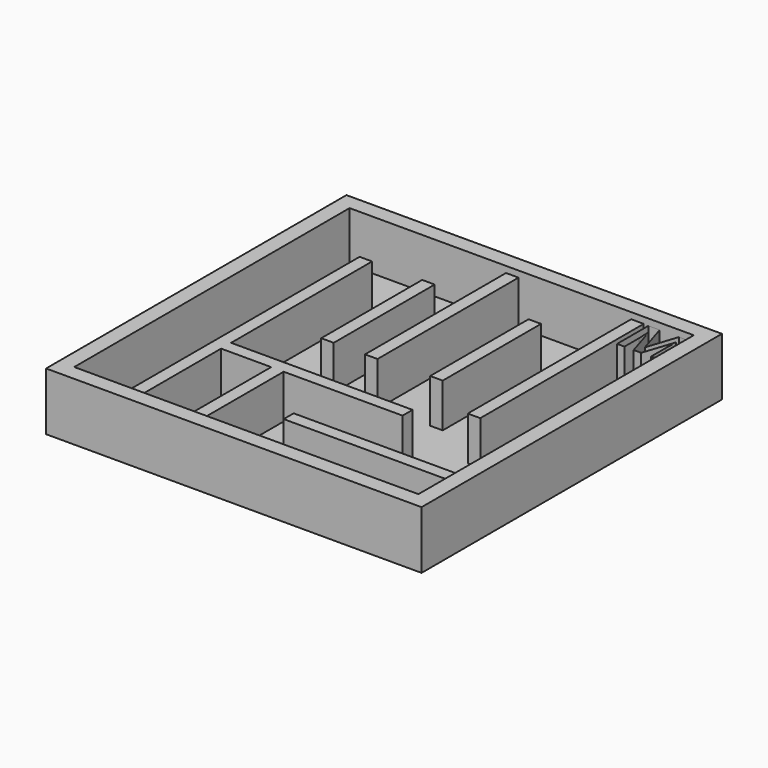
from build123d import *

# Parameters (mm, degrees)
F0_W         = 38.1
F0_H         = 38.1
F1_DEPTH     = 0.79375
F2_W         = 38.1
F2_H         = 38.1
F2_W_2       = 34.925
F2_H_2       = 34.925
F3_DEPTH     = 5.08
F4_W         = 1.27
F4_H         = 12.8048420015
F4_H_2       = 17.8848420015
F4_H_3       = 12.4767818307
F4_H_4       = 20.7282226267
F4_W_2       = 17.145
F4_H_5       = 1.27
F5_DEPTH     = 4.445
F4_TEXT_SIZE = 5.5579939571
F6_DEPTH     = 4.445
F4_R         = 1.27
F7_DEPTH     = 0.396875


# Not quite as in the source:
# - Text() gives the source's letters only with a copy of the font that has no kerning and outlines rounded to 1/6400 em; it was checked with that copy


with BuildPart() as f1:
    # F0 (on Top) → F1 (new body)
    with BuildSketch(Plane.XY):
        with Locations((-1.3391338289, 1.1490499321)):
            Rectangle(F0_W, F0_H)
    extrude(amount=F1_DEPTH)

    # F2 (on face) → F3 (join)
    with BuildSketch(Plane.XY.offset(0.79375)):
        with Locations((-1.3391338289, 1.1490499321)):
            Rectangle(F2_W, F2_H)
        with Locations((-1.3391338289, 1.1490499321)):
            Rectangle(F2_W_2, F2_H_2, mode=Mode.SUBTRACT)
    extrude(amount=F3_DEPTH)

    # F4 (on face) → F5 (join)
    with BuildSketch(Plane.XY.offset(0.79375)):
        Polygon((-13.7216338289, -16.3134500679), (-12.4516338289, -16.3134500679), (-12.4516338289, -5.6232920694), (-7.3716338289, -5.6232920694), (-7.3716338289, -16.3134500679), (-6.1016338289, -16.3134500679), (-6.1016338289, -5.6232920694), (5.9633661711, -5.6232920694), (5.9633661711, -4.3532920694), (-12.4516338289, -4.3532920694), (-12.4516338289, 13.5315499321), (-13.7216338289, 13.5315499321), align=None)
        with Locations((-6.7366338289, 7.1291289313)):
            Rectangle(F4_W, F4_H)
        with Locations((-2.2916338289, 9.6691289313)):
            Rectangle(F4_W, F4_H_2)
        with Locations((4.0583661711, 7.2931590167)):
            Rectangle(F4_W, F4_H_3)
        with Locations((10.4083661711, 8.2474386187)):
            Rectangle(F4_W, F4_H_4)
        with Locations((7.5508661711, -11.3382920694)):
            Rectangle(F4_W_2, F4_H_5)
    extrude(amount=F5_DEPTH)

    # F4 (on face) → F6 (join)
    with BuildSketch(Plane.XY.offset(0.79375)):
        with Locations((11.0433661711, 14.6097942829)):
            Text('M', F4_TEXT_SIZE, font='Open Sans', font_style=FontStyle.BOLD, text_align=(TextAlign.LEFT, TextAlign.BOTTOM))
    extrude(amount=F6_DEPTH)

    # F4 (on face) → F7 (cut)
    with BuildSketch(Plane.XY.offset(0.79375)):
        with Locations((-16.2616338289, -12.2631704435)):
            Circle(F4_R)
        with Locations((12.3133661711, -13.9391720295)):
            Circle(F4_R)
    extrude(amount=-F7_DEPTH, mode=Mode.SUBTRACT)


solid = f1.part
